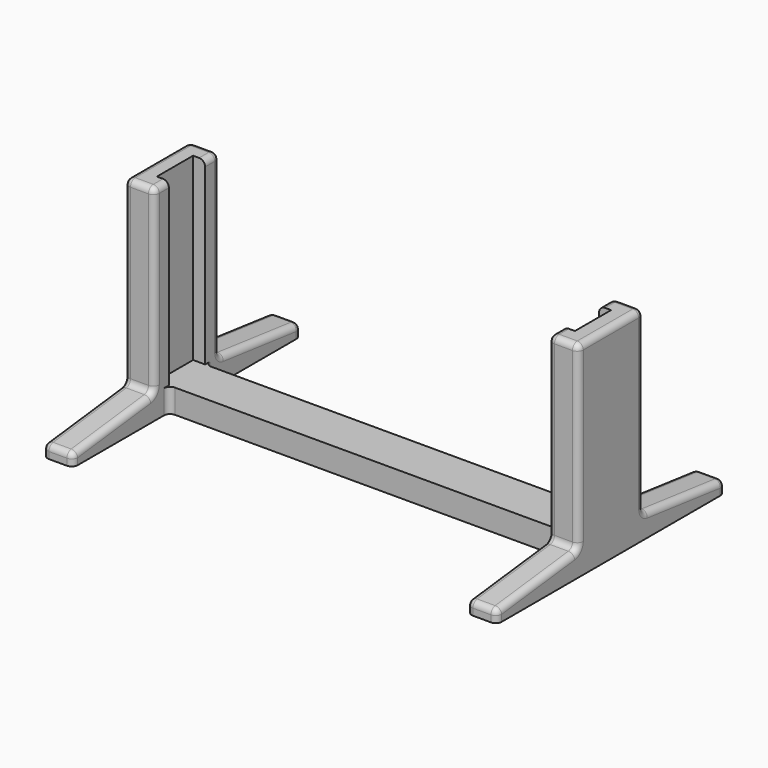
from build123d import *

# Parameters (mm, degrees)
F0_W     = 5
F0_H     = 17
F0_W_2   = 3
F0_H_2   = 7.55
F1_DEPTH = 4
F2_DEPTH = 30
F4_DEPTH = 75.711
F5_R     = 1


with BuildPart() as f1:
    # F0 (on Top) → F1 (new body)
    with BuildSketch(Plane.XY):
        with Locations((-35.355, 15.275)):
            Rectangle(F0_W, F0_H)
        Polygon((-34.855, 3.775), (-32.855, 3.775), (-32.855, 6.775), (-37.855, 6.775), (-37.855, 3.775), align=None)
        with Locations((-35.355, -15.275)):
            Rectangle(F0_W, F0_H)
        Polygon((37.855, -3.775), (34.855, -3.775), (32.855, -3.775), (32.855, -6.775), (37.855, -6.775), align=None)
        with Locations((35.355, 15.275)):
            Rectangle(F0_W, F0_H)
        with Locations((-36.355, 0)):
            Rectangle(F0_W_2, F0_H_2)
        Polygon((-32.855, -6.775), (-32.855, -3.775), (-34.855, -3.775), (-37.855, -3.775), (-37.855, -6.775), align=None)
        Polygon((32.855, -3.775), (34.855, -3.775), (34.855, 3.775), (32.855, 3.775), (-32.855, 3.775), (-34.855, 3.775), (-34.855, -3.775), (-32.855, -3.775), align=None)
        with Locations((36.355, 0)):
            Rectangle(F0_W_2, F0_H_2)
        Polygon((32.855, 3.775), (34.855, 3.775), (37.855, 3.775), (37.855, 6.775), (32.855, 6.775), align=None)
        with Locations((35.355, -15.275)):
            Rectangle(F0_W, F0_H)
    extrude(amount=-F1_DEPTH)

    # F0 (on Top) → F2 (join)
    with BuildSketch(Plane.XY):
        Polygon((-34.855, 3.775), (-32.855, 3.775), (-32.855, 6.775), (-37.855, 6.775), (-37.855, 3.775), align=None)
        with Locations((-36.355, 0)):
            Rectangle(F0_W_2, F0_H_2)
        Polygon((-32.855, -6.775), (-32.855, -3.775), (-34.855, -3.775), (-37.855, -3.775), (-37.855, -6.775), align=None)
        Polygon((32.855, 3.775), (34.855, 3.775), (37.855, 3.775), (37.855, 6.775), (32.855, 6.775), align=None)
        with Locations((36.355, 0)):
            Rectangle(F0_W_2, F0_H_2)
        Polygon((37.855, -3.775), (34.855, -3.775), (32.855, -3.775), (32.855, -6.775), (37.855, -6.775), align=None)
    extrude(amount=F2_DEPTH)

    # F3 (on face) → F4 (cut, through all)
    with BuildSketch(Plane.YZ.offset(37.855)):
        Polygon((-23.775, -2), (-6.775, 0), (-23.775, 0), align=None)
        Polygon((23.775, 0), (6.775, 0), (23.775, -2), align=None)
    extrude(amount=-F4_DEPTH, mode=Mode.SUBTRACT)

    # F5
    f5_edges = [f1.edges().sort_by_distance(p)[0] for p in [
        (-37.855, 0, 30),
        (-35.355, -6.775, 30),
        (-37.855, -6.775, 15),
        (35.355, -6.775, 30),
        (37.855, 0, 30),
        (37.855, -6.775, 15),
        (37.855, -15.275, -1),
        (35.355, -23.775, -2),
        (37.855, -23.775, -3),
        (32.855, -23.775, -3),
        (32.855, -15.275, -1),
        (32.855, -6.775, 15),
        (-35.355, -23.775, -2),
        (-37.855, -23.775, -3),
        (-32.855, -23.775, -3),
        (-37.855, -15.275, -1),
        (-32.855, -15.275, -1),
        (-32.855, -6.775, 15),
        (-32.855, -5.275, 30),
        (32.855, -5.275, 30),
        (35.355, 6.775, 30),
        (37.855, 6.775, 15),
        (35.355, -6.775, 0),
        (-35.355, -6.775, 0),
        (35.355, 6.775, 0),
        (37.855, 15.275, -1),
        (35.355, 23.775, -2),
        (32.855, 15.275, -1),
        (37.855, 23.775, -3),
        (32.855, 23.775, -3),
        (-32.855, 15.275, -1),
        (-35.355, 23.775, -2),
        (-37.855, 15.275, -1),
        (-35.355, 6.775, 0),
        (-35.355, 6.775, 30),
        (-32.855, 5.275, 30),
        (-32.855, 23.775, -3),
        (-37.855, 23.775, -3),
        (-32.855, -3.775, -2),
        (32.855, -3.775, -2),
        (-32.855, 3.775, -2),
        (32.855, 3.775, -2),
        (32.855, 5.275, 30),
        (-37.855, 6.775, 15),
        (-32.855, 6.775, 15),
        (32.855, 6.775, 15),
    ]]
    fillet(f5_edges, radius=F5_R)


solid = f1.part
